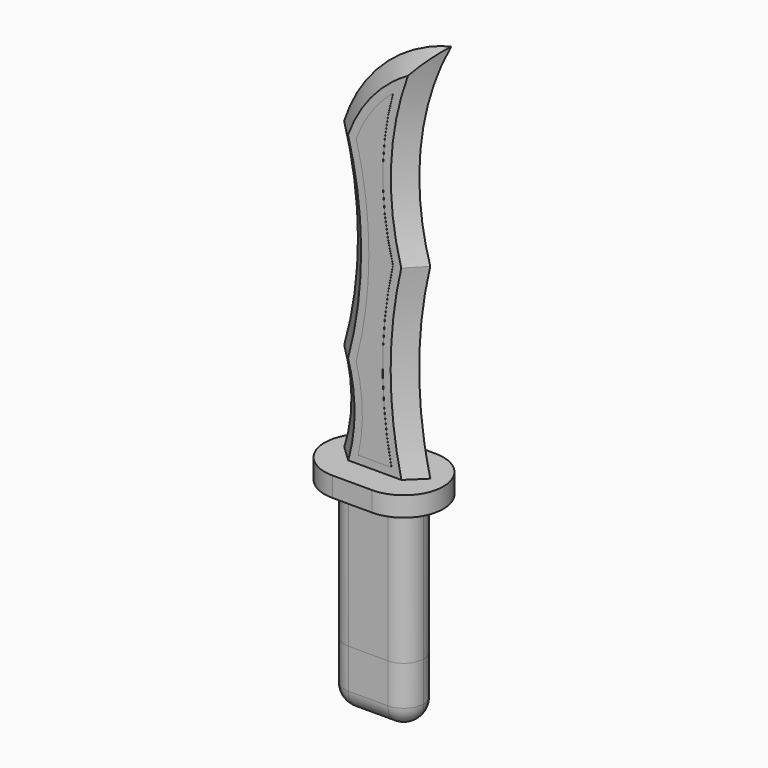
from build123d import *

# Parameters (mm, degrees)
F0_W         = 20
F0_H         = 35
F1_DEPTH     = 10
F0_H_2       = 15
F2_DEPTH     = 10
F3_R         = 4.99999
F3_2_R       = 4.99999
F5_DEPTH     = 5
F6_DEPTH     = 8
F7_SIZE      = 7
F8_T2_ANGLE  = 84.342415
F8_T4_ANGLE  = 49.305112
F9_C1_SIZE   = 7
F9_C2_SIZE   = 7
F9_C3_SIZE   = 7
F10_T2_ANGLE = 101.756181
F10_T4_ANGLE = 56.431155
F10_T6_ANGLE = 105.999601
F12_DEPTH    = 0.05
F14_DEPTH    = 0.05


# Not quite as in the source:
# - a fillet or chamfer that OpenCascade refuses, or shapes differently, is made with other operations: its cross-section is extruded or revolved along the edge and cut away or added
# - a fillet or chamfer is up to 0.001 mm smaller than in the source, because OpenCascade refuses the exact size


with BuildPart() as f1:
    # F0 (on Front) → F1 (new body)
    with BuildSketch(Plane.XZ):
        with Locations((0.076923, -17.5)):
            Rectangle(F0_W, F0_H)
    extrude(amount=F1_DEPTH)

    # F3 (radius 5 in the source; OpenCascade refuses exactly that, so slightly less here)
    f3_edges = [f1.edges().sort_by_distance(p)[0] for p in [
        (10.076923, -10, -17.5),
        (10.076923, 0, -17.5),
        (-9.923077, 0, -17.5),
        (-9.923077, -10, -17.5),
    ]]
    fillet(f3_edges, radius=F3_R)


with BuildPart() as f2:
    # F0 (on Front) → F2 (new body)
    with BuildSketch(Plane.XZ):
        with Locations((0.076923, -42.5)):
            Rectangle(F0_W, F0_H_2)
    extrude(amount=F2_DEPTH)

    # F3#2 (radius 5 in the source; OpenCascade refuses exactly that, so slightly less here)
    f3_2_edges = [f2.edges().sort_by_distance(p)[0] for p in [
        (10.076923, -10, -42.5),
        (10.076923, 0, -42.5),
        (-9.923077, 0, -42.5),
        (-9.923077, -10, -42.5),
        (0.076923, -10, -50),
        (-9.923077, -5, -50),
        (0.076923, 0, -50),
        (10.076923, -5, -50),
    ]]
    fillet(f3_2_edges, radius=F3_2_R)


with BuildPart() as f5:
    # F4 (on Top) → F5 (new body)
    with BuildSketch(Plane.XY):
        with BuildLine():
            Line((-4.923077, -15), (5.076923, -15))
            ThreePointArc((5.076923, -15), (15.076923, -5), (5.076923, 5))
            Line((5.076923, 5), (-4.923077, 5))
            ThreePointArc((-4.923077, 5), (-14.923077, -5), (-4.923077, -15))
        make_face()
    extrude(amount=F5_DEPTH)


with BuildPart() as f6:
    # F0 (on Front) → F6 (new body)
    with BuildSketch(Plane.XZ):
        with BuildLine():
            ThreePointArc((-13.923077, 27.566807), (-11.949291, 16.283404), (-13.923077, 5))
            Line((-13.923077, 5), (14.076923, 5))
            ThreePointArc((14.076923, 5), (11.159544, 28.657342), (14.076923, 52.314684))
            ThreePointArc((14.076923, 52.314684), (11.898675, 80.51991), (22.238776, 106.851675))
            ThreePointArc((22.238776, 106.851675), (-0.401041, 97.806903), (-13.923077, 77.520855))
            ThreePointArc((-13.923077, 77.520855), (-10.303353, 52.543831), (-13.923077, 27.566807))
        make_face()
    extrude(amount=F6_DEPTH)

    # F7
    f7_edges = [f6.edges().sort_by_distance(p)[0] for p in [
        (11.898675, -8, 80.51991),
        (11.159544, -8, 28.657342),
    ]]
    chamfer(f7_edges, length=F7_SIZE)

    # F8: chamfer of 7 on 2 edges, made by hand

    # F8_s1 → F8_t2 (revolve, cut)
    with BuildSketch(Plane(origin=(-9.96544, 0, 14.965368), x_dir=(0, 1, 0), z_dir=(0.554258, 0, -0.832345))):
        Polygon((0, 31.166494), (-7, 38.166494), (0, 38.166494), align=None)
    revolve(axis=Axis((74.426742, 0, 71.162134), (0, 1, 0)), revolution_arc=F8_T2_ANGLE, mode=Mode.SUBTRACT)

    # F8_s3 → F8_t4 (revolve, cut)
    with BuildSketch(Plane(origin=(8.020087, 0, -17.475022), x_dir=(0, 1, 0), z_dir=(0.417115, 0, -0.908854))):
        Polygon((-7, 13.220105), (0, 6.220105), (0, 13.220105), align=None)
    revolve(axis=Axis((108.538203, 0, 28.657342), (0, 1, 0)), revolution_arc=F8_T4_ANGLE, mode=Mode.SUBTRACT)

    # F9: chamfer of 7 on 3 edges, made by hand

    # F9_c1
    f9_c1_edges = [f6.edges().sort_by_distance(p)[0] for p in [
        (-11.949291, 0, 16.283404),
    ]]
    chamfer(f9_c1_edges, length=F9_C1_SIZE)

    # F9_c2
    f9_c2_edges = [f6.edges().sort_by_distance(p)[0] for p in [
        (-10.474122, 0, 58.022937),
    ]]
    chamfer(f9_c2_edges, length=F9_C2_SIZE)

    # F9_c3
    f9_c3_edges = [f6.edges().sort_by_distance(p)[0] for p in [
        (-0.077753, 0, 98.066427),
    ]]
    chamfer(f9_c3_edges, length=F9_C3_SIZE)

    # F10: chamfer of 7 on 3 edges, made by hand

    # F10_s1 → F10_t2 (revolve, cut)
    with BuildSketch(Plane(origin=(-35.168204, 0, 28.602761), x_dir=(0, 1, 0), z_dir=(-0.775805, 0, 0.630973))):
        with BuildLine():
            Line((-0.80201, -17.160971), (-8.19799, -24.556951))
            Line((-8.19799, -24.556951), (-8.33799, -24.556951))
            ThreePointArc((-8.33799, -24.556951), (-8.14, -20.957956), (-8.14, -17.358961))
            Line((-8.14, -17.358961), (-8, -17.218961))
            ThreePointArc((-8, -17.218961), (-4.401005, -17.218961), (-0.80201, -17.020971))
            Line((-0.80201, -17.020971), (-0.80201, -17.160971))
        make_face()
    revolve(axis=Axis((-45.187699, -8, 16.283404), (0, 1, 0)), revolution_arc=F10_T2_ANGLE, mode=Mode.SUBTRACT)

    # F10_s3 → F10_t4 (revolve, cut)
    with BuildSketch(Plane(origin=(-43.860537, 0, 81.746181), x_dir=(0, 1, 0), z_dir=(-0.47279, 0, 0.881175))):
        with BuildLine():
            Line((-0.80201, -26.01985), (-8.19799, -33.41583))
            Line((-8.19799, -33.41583), (-8.33799, -33.41583))
            ThreePointArc((-8.33799, -33.41583), (-8.14, -29.816835), (-8.14, -26.21784))
            Line((-8.14, -26.21784), (-8, -26.07784))
            ThreePointArc((-8, -26.07784), (-4.401005, -26.07784), (-0.80201, -25.87985))
            Line((-0.80201, -25.87985), (-0.80201, -26.01985))
        make_face()
    revolve(axis=Axis((-98.287153, -8, 52.543831), (0, 1, 0)), revolution_arc=F10_T4_ANGLE, mode=Mode.SUBTRACT)

    # F10_s5 → F10_t6 (revolve, cut)
    with BuildSketch(Plane(origin=(16.752884, 0, -2.144949), x_dir=(0, 1, 0), z_dir=(0.991903, 0, -0.126998))):
        with BuildLine():
            Line((-0.80201, 109.877266), (-8.19799, 102.481286))
            Line((-8.19799, 102.481286), (-8.33799, 102.481286))
            ThreePointArc((-8.33799, 102.481286), (-8.14, 106.080281), (-8.14, 109.679276))
            Line((-8.14, 109.679276), (-8, 109.819276))
            ThreePointArc((-8, 109.819276), (-4.401005, 109.819276), (-0.80201, 110.017266))
            Line((-0.80201, 110.017266), (-0.80201, 109.877266))
        make_face()
    revolve(axis=Axis((25.466846, -8, 65.914486), (0, -1, 0)), revolution_arc=F10_T6_ANGLE, mode=Mode.SUBTRACT)


with BuildPart() as f12:
    # F11 (on face) → F12 (new body)
    with BuildSketch(Plane.XZ.offset(8)):
        with BuildLine():
            Line((-3.982098, 7), (4.387453, 7))
            ThreePointArc((4.387453, 7), (2.163365, 29.558998), (4.769536, 52.077054))
            ThreePointArc((4.769536, 52.077054), (2.202401, 71.268091), (4.825833, 90.451512))
            ThreePointArc((4.825833, 90.451512), (-0.68537, 84.46654), (-4.512815, 77.28713))
            ThreePointArc((-4.512815, 77.28713), (-1.30336, 52.508848), (-4.530689, 27.732888))
            ThreePointArc((-4.530689, 27.732888), (-2.964069, 17.400639), (-3.982098, 7))
        make_face()
    extrude(amount=F12_DEPTH)


with BuildPart() as f14:
    # F13 (on face) → F14 (new body)
    with BuildSketch(Plane(origin=(0, 0, 0), x_dir=(-1, 0, 0), z_dir=(0, 1, 0))):
        with BuildLine():
            ThreePointArc((-4.825833, 90.451512), (-2.202401, 71.268091), (-4.769536, 52.077054))
            ThreePointArc((-4.769536, 52.077054), (-2.163365, 29.558998), (-4.387453, 7))
            Line((-4.387453, 7), (3.982098, 7))
            ThreePointArc((3.982098, 7), (2.964069, 17.400639), (4.530689, 27.732888))
            ThreePointArc((4.530689, 27.732888), (1.30336, 52.508848), (4.512815, 77.28713))
            ThreePointArc((4.512815, 77.28713), (0.68537, 84.46654), (-4.825833, 90.451512))
        make_face()
    extrude(amount=F14_DEPTH)


solid = Compound([f1.part, f2.part, f5.part, f6.part, f12.part, f14.part])
